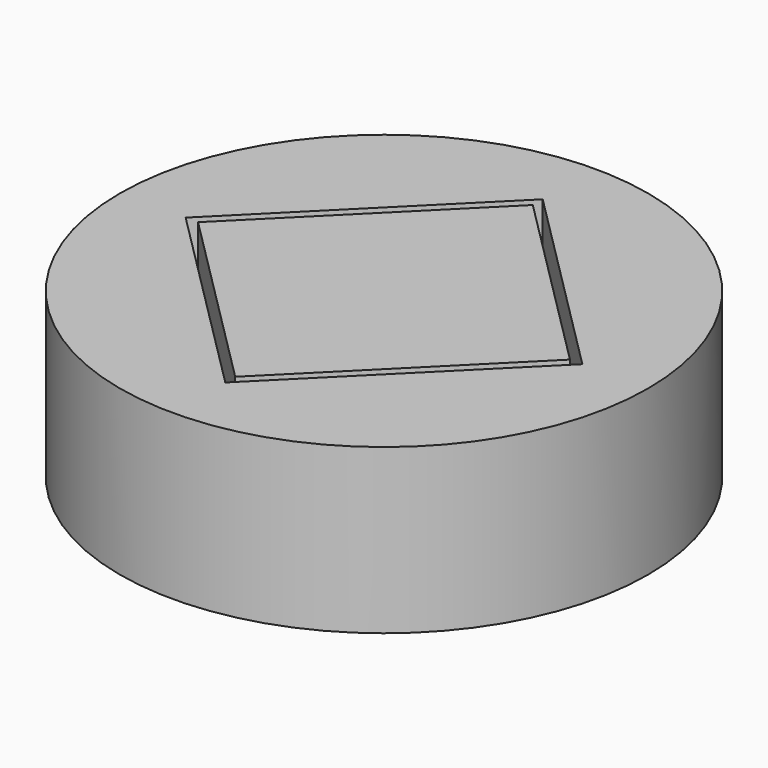
from build123d import *

# Parameters (mm, degrees)
F1_DEPTH = 37.4
F2_R     = 4.8964779363
F3_DEPTH = 55.6
F4_R     = 60.2548339959
F5_DEPTH = 37.4


with BuildPart() as f1:
    # F0 (on Top) → F1 (new body)
    with BuildSketch(Plane.XY):
        Polygon((0, 42.4264068712), (-42.4264068712, 0), (0, -42.4264068712), (42.4264068712, 0), align=None)
    extrude(amount=F1_DEPTH)

    # F2 (on face) → F3 (cut)
    with BuildSketch(Plane(origin=(-21.2132034356, -21.2132034356, 0), x_dir=(0.7071067812, -0.7071067812, 0), z_dir=(-0.7071067812, -0.7071067812, 0))):
        with Locations((0, 20.5192621797)):
            Circle(F2_R)
    extrude(amount=-F3_DEPTH, mode=Mode.SUBTRACT)


with BuildPart() as f5:
    # F4 (on Top) → F5 (new body, through all)
    with BuildSketch(Plane.XY):
        Circle(F4_R)
        Polygon((45.2548339959, 0), (0, -45.2548339959), (-45.2548339959, 0), (0, 45.2548339959), align=None, mode=Mode.SUBTRACT)
    extrude(amount=F5_DEPTH)


solid = Compound([f1.part, f5.part])
